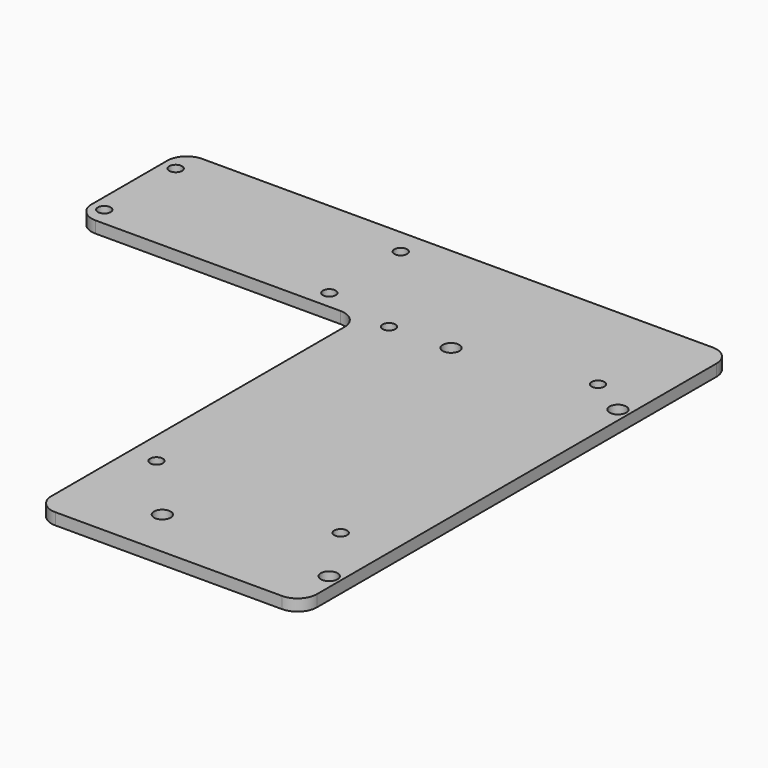
from build123d import *

# Parameters (mm, degrees)
F1_DEPTH = 3
F2_D     = 3.3
F3_D     = 4.3
F4_R     = 5


# Not quite as in the source:
# - a feature names something its author has since deleted; it is built from what else it names


with BuildPart() as f1:
    # F0 (on Top) → F1 (new body)
    with BuildSketch(Plane.XY):
        Polygon((-43.9476147294, -59.139739722), (24.4538411498, -59.139739722), (24.4538411498, 79.5589722693), (-117.0655786991, 79.5589722693), (-117.0655786991, 45.1967306435), (-43.9476147294, 45.1967306435), align=None)
    extrude(amount=F1_DEPTH)

    # F2 (through all)
    with Locations(Plane(origin=(0, 0, 0), x_dir=(1, 0, 0), z_dir=(0, 0, -1))):
        with Locations((-113.6049106717, -72.9293674231), (-113.6049106717, -49.9293674231), (-55.6049106717, -49.9293674231), (-55.6049106717, -72.9293674231), (-37.0104938323, -45.9071589798), (11.4895061677, -52.6071589798), (11.4895061677, 30.2928410202), (-37.0104938323, 28.9928410202)):
            Hole(F2_D / 2)

    # F3 (through all)
    with Locations(Plane(origin=(0, 0, 0), x_dir=(1, 0, 0), z_dir=(0, 0, -1))):
        with Locations((-21.5, -46.5), (21.5, -46.5), (21.5, 46.5), (-21.5, 46.5)):
            Hole(F3_D / 2)

    # F4
    f4_edges = [f1.edges().sort_by_distance(p)[0] for p in [
        (-117.065579, 79.558972, 1.5),
        (-43.947615, 45.196731, 1.5),
        (-117.065579, 45.196731, 1.5),
        (24.453841, 79.558972, 1.5),
        (24.453841, -59.13974, 1.5),
        (-43.947615, -59.13974, 1.5),
    ]]
    fillet(f4_edges, radius=F4_R)


solid = f1.part
